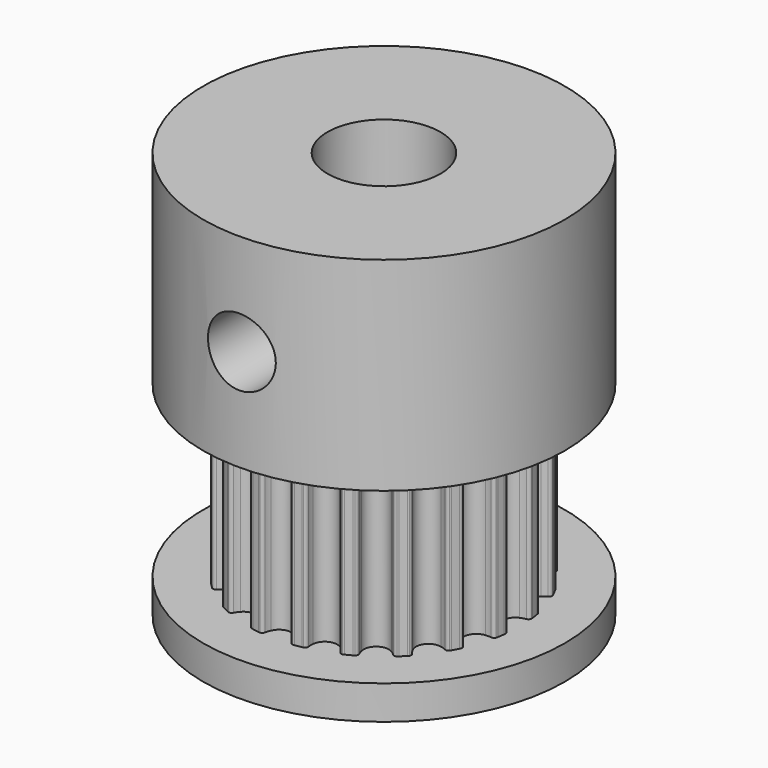
from build123d import *

# Parameters (mm, degrees)
F1_DEPTH  = 7.5
F2_R      = 8
F3_DEPTH  = 9
F4_R      = 8
F5_DEPTH  = 1.5
F6_R      = 2.5
F7_DEPTH  = 18.001
F8_R      = 1.5
F9_DEPTH  = 8.001
F10_R     = 1.5
F11_DEPTH = 10


with BuildPart() as f1:
    # F0 (on Top) → F1 (new body)
    with BuildSketch(Plane.XY):
        with BuildLine():
            ThreePointArc((-0.5137469529, -5.5950260293), (0, -5.25), (0.5137469529, -5.5950260293))
            ThreePointArc((0.5137469529, -5.5950260293), (0.5592692601, -5.7125893356), (0.5896381917, -5.8349459432))
            ThreePointArc((0.5896381917, -5.8349459432), (0.634011817, -5.9169199806), (0.718236871, -5.9568562008))
            ThreePointArc((0.718236871, -5.9568562008), (0.7555100891, -5.952243653), (0.7927537045, -5.9473978818))
            ThreePointArc((0.7927537045, -5.9473978818), (0.9386067902, -5.9261300436), (1.0838934413, -5.9012858775))
            ThreePointArc((1.0838934413, -5.9012858775), (1.1208116501, -5.8943855698), (1.1576859427, -5.8872543055))
            ThreePointArc((1.1576859427, -5.8872543055), (1.2254477584, -5.82324573), (1.2423182132, -5.7315715833))
            ThreePointArc((1.2423182132, -5.7315715833), (1.2333905124, -5.6058190183), (1.2403557397, -5.4799425032))
            ThreePointArc((1.2403557397, -5.4799425032), (1.6223392205, -4.9930467105), (2.2175605143, -5.1624294247))
            ThreePointArc((2.2175605143, -5.1624294247), (2.2971838607, -5.2601716067), (2.3638767022, -5.3671551397))
            ThreePointArc((2.3638767022, -5.3671551397), (2.4314098983, -5.4314048778), (2.5238536555, -5.4433595073))
            ThreePointArc((2.5238536555, -5.4433595073), (2.5578772368, -5.4274546558), (2.5918005942, -5.4113371434))
            ThreePointArc((2.5918005942, -5.4113371434), (2.7239429984, -5.3460391451), (2.8544415451, -5.2775148949))
            ThreePointArc((2.8544415451, -5.2775148949), (2.8874205358, -5.2595439583), (2.9202863902, -5.2413669399))
            ThreePointArc((2.9202863902, -5.2413669399), (2.964951969, -5.1595516144), (2.9526678557, -5.0671510626))
            ThreePointArc((2.9526678557, -5.0671510626), (2.905317428, -4.9503120775), (2.8730437705, -4.828444024))
            ThreePointArc((2.8730437705, -4.828444024), (3.0858725745, -4.2473392205), (3.7043038019, -4.2244982593))
            ThreePointArc((3.7043038019, -4.2244982593), (3.8102340997, -4.2928516312), (3.906722491, -4.373989796))
            ThreePointArc((3.906722491, -4.373989796), (3.9908046381, -4.4142260228), (4.0824180595, -4.3970288591))
            ThreePointArc((4.0824180595, -4.3970288591), (4.1098615388, -4.3713885816), (4.1371439837, -4.3455770225))
            ThreePointArc((4.1371439837, -4.3455770225), (4.2426406871, -4.2426406871), (4.3455770225, -4.1371439837))
            ThreePointArc((4.3455770225, -4.1371439837), (4.3713885816, -4.1098615388), (4.3970288591, -4.0824180595))
            ThreePointArc((4.3970288591, -4.0824180595), (4.4142260228, -3.9908046381), (4.373989796, -3.906722491))
            ThreePointArc((4.373989796, -3.906722491), (4.2928516312, -3.8102340997), (4.2244982593, -3.7043038019))
            ThreePointArc((4.2244982593, -3.7043038019), (4.2473392205, -3.0858725745), (4.828444024, -2.8730437705))
            ThreePointArc((4.828444024, -2.8730437705), (4.9503120775, -2.905317428), (5.0671510626, -2.9526678557))
            ThreePointArc((5.0671510626, -2.9526678557), (5.1595516144, -2.964951969), (5.2413669399, -2.9202863902))
            ThreePointArc((5.2413669399, -2.9202863902), (5.2595439583, -2.8874205358), (5.2775148949, -2.8544415451))
            ThreePointArc((5.2775148949, -2.8544415451), (5.3460391451, -2.7239429984), (5.4113371434, -2.5918005942))
            ThreePointArc((5.4113371434, -2.5918005942), (5.4432427829, -2.4673716464), (5.3671551397, -2.3638767022))
            ThreePointArc((5.3671551397, -2.3638767022), (5.2601716067, -2.2971838607), (5.1624294247, -2.2175605143))
            ThreePointArc((5.1624294247, -2.2175605143), (4.9930467105, -1.6223392205), (5.4799425032, -1.2403557397))
            ThreePointArc((5.4799425032, -1.2403557397), (5.6058190183, -1.2333905124), (5.7315715833, -1.2423182132))
            ThreePointArc((5.7315715833, -1.2423182132), (5.82324573, -1.2254477584), (5.8872543055, -1.1576859427))
            ThreePointArc((5.8872543055, -1.1576859427), (5.8943855698, -1.1208116501), (5.9012858775, -1.0838934413))
            ThreePointArc((5.9012858775, -1.0838934413), (5.9261300436, -0.9386067902), (5.9473978818, -0.7927537045))
            ThreePointArc((5.9473978818, -0.7927537045), (5.952243653, -0.7555100891), (5.9568562008, -0.718236871))
            ThreePointArc((5.9568562008, -0.718236871), (5.9169199806, -0.634011817), (5.8349459432, -0.5896381917))
            ThreePointArc((5.8349459432, -0.5896381917), (5.7125893356, -0.5592692601), (5.5950260293, -0.5137469529))
            ThreePointArc((5.5950260293, -0.5137469529), (5.25, 0), (5.5950260293, 0.5137469529))
            ThreePointArc((5.5950260293, 0.5137469529), (5.7125893356, 0.5592692601), (5.8349459432, 0.5896381917))
            ThreePointArc((5.8349459432, 0.5896381917), (5.9169199806, 0.634011817), (5.9568562008, 0.718236871))
            ThreePointArc((5.9568562008, 0.718236871), (5.952243653, 0.7555100891), (5.9473978818, 0.7927537045))
            ThreePointArc((5.9473978818, 0.7927537045), (5.9261300436, 0.9386067902), (5.9012858775, 1.0838934413))
            ThreePointArc((5.9012858775, 1.0838934413), (5.8943855698, 1.1208116501), (5.8872543055, 1.1576859427))
            ThreePointArc((5.8872543055, 1.1576859427), (5.82324573, 1.2254477584), (5.7315715833, 1.2423182132))
            ThreePointArc((5.7315715833, 1.2423182132), (5.6058190183, 1.2333905124), (5.4799425032, 1.2403557397))
            ThreePointArc((5.4799425032, 1.2403557397), (4.9930467105, 1.6223392205), (5.1624294247, 2.2175605143))
            ThreePointArc((5.1624294247, 2.2175605143), (5.2601716067, 2.2971838607), (5.3671551397, 2.3638767022))
            ThreePointArc((5.3671551397, 2.3638767022), (5.4314048778, 2.4314098983), (5.4433595073, 2.5238536555))
            ThreePointArc((5.4433595073, 2.5238536555), (5.4274546558, 2.5578772368), (5.4113371434, 2.5918005942))
            ThreePointArc((5.4113371434, 2.5918005942), (5.3460391451, 2.7239429984), (5.2775148949, 2.8544415451))
            ThreePointArc((5.2775148949, 2.8544415451), (5.2595439583, 2.8874205358), (5.2413669399, 2.9202863902))
            ThreePointArc((5.2413669399, 2.9202863902), (5.1595516144, 2.964951969), (5.0671510626, 2.9526678557))
            ThreePointArc((5.0671510626, 2.9526678557), (4.9503120775, 2.905317428), (4.828444024, 2.8730437705))
            ThreePointArc((4.828444024, 2.8730437705), (4.2473392205, 3.0858725745), (4.2244982593, 3.7043038019))
            ThreePointArc((4.2244982593, 3.7043038019), (4.2928516312, 3.8102340997), (4.373989796, 3.906722491))
            ThreePointArc((4.373989796, 3.906722491), (4.4142260228, 3.9908046381), (4.3970288591, 4.0824180595))
            ThreePointArc((4.3970288591, 4.0824180595), (4.3713885816, 4.1098615388), (4.3455770225, 4.1371439837))
            ThreePointArc((4.3455770225, 4.1371439837), (4.2426406871, 4.2426406871), (4.1371439837, 4.3455770225))
            ThreePointArc((4.1371439837, 4.3455770225), (4.1098615388, 4.3713885816), (4.0824180595, 4.3970288591))
            ThreePointArc((4.0824180595, 4.3970288591), (3.9908046381, 4.4142260228), (3.906722491, 4.373989796))
            ThreePointArc((3.906722491, 4.373989796), (3.8102340997, 4.2928516312), (3.7043038019, 4.2244982593))
            ThreePointArc((3.7043038019, 4.2244982593), (3.0858725745, 4.2473392205), (2.8730437705, 4.828444024))
            ThreePointArc((2.8730437705, 4.828444024), (2.905317428, 4.9503120775), (2.9526678557, 5.0671510626))
            ThreePointArc((2.9526678557, 5.0671510626), (2.964951969, 5.1595516144), (2.9202863902, 5.2413669399))
            ThreePointArc((2.9202863902, 5.2413669399), (2.8874205358, 5.2595439583), (2.8544415451, 5.2775148949))
            ThreePointArc((2.8544415451, 5.2775148949), (2.7239429984, 5.3460391451), (2.5918005942, 5.4113371434))
            ThreePointArc((2.5918005942, 5.4113371434), (2.5578772368, 5.4274546558), (2.5238536555, 5.4433595073))
            ThreePointArc((2.5238536555, 5.4433595073), (2.4314098983, 5.4314048778), (2.3638767022, 5.3671551397))
            ThreePointArc((2.3638767022, 5.3671551397), (2.2971838607, 5.2601716067), (2.2175605143, 5.1624294247))
            ThreePointArc((2.2175605143, 5.1624294247), (1.6223392205, 4.9930467105), (1.2403557397, 5.4799425032))
            ThreePointArc((1.2403557397, 5.4799425032), (1.2333905124, 5.6058190183), (1.2423182132, 5.7315715833))
            ThreePointArc((1.2423182132, 5.7315715833), (1.2254477584, 5.82324573), (1.1576859427, 5.8872543055))
            ThreePointArc((1.1576859427, 5.8872543055), (1.1208116501, 5.8943855698), (1.0838934413, 5.9012858775))
            ThreePointArc((1.0838934413, 5.9012858775), (0.9386067902, 5.9261300436), (0.7927537045, 5.9473978818))
            ThreePointArc((0.7927537045, 5.9473978818), (0.7555100891, 5.952243653), (0.718236871, 5.9568562008))
            ThreePointArc((0.718236871, 5.9568562008), (0.634011817, 5.9169199806), (0.5896381917, 5.8349459432))
            ThreePointArc((0.5896381917, 5.8349459432), (0.5592692601, 5.7125893356), (0.5137469529, 5.5950260293))
            ThreePointArc((0.5137469529, 5.5950260293), (0, 5.25), (-0.5137469529, 5.5950260293))
            ThreePointArc((-0.5137469529, 5.5950260293), (-0.5592692601, 5.7125893356), (-0.5896381917, 5.8349459432))
            ThreePointArc((-0.5896381917, 5.8349459432), (-0.634011817, 5.9169199806), (-0.718236871, 5.9568562008))
            ThreePointArc((-0.718236871, 5.9568562008), (-0.7555100891, 5.952243653), (-0.7927537045, 5.9473978818))
            ThreePointArc((-0.7927537045, 5.9473978818), (-0.9386067902, 5.9261300436), (-1.0838934413, 5.9012858775))
            ThreePointArc((-1.0838934413, 5.9012858775), (-1.1208116501, 5.8943855698), (-1.1576859427, 5.8872543055))
            ThreePointArc((-1.1576859427, 5.8872543055), (-1.2254477584, 5.82324573), (-1.2423182132, 5.7315715833))
            ThreePointArc((-1.2423182132, 5.7315715833), (-1.2333905124, 5.6058190183), (-1.2403557397, 5.4799425032))
            ThreePointArc((-1.2403557397, 5.4799425032), (-1.6223392205, 4.9930467105), (-2.2175605143, 5.1624294247))
            ThreePointArc((-2.2175605143, 5.1624294247), (-2.2971838607, 5.2601716067), (-2.3638767022, 5.3671551397))
            ThreePointArc((-2.3638767022, 5.3671551397), (-2.4314098983, 5.4314048778), (-2.5238536555, 5.4433595073))
            ThreePointArc((-2.5238536555, 5.4433595073), (-2.5578772368, 5.4274546558), (-2.5918005942, 5.4113371434))
            ThreePointArc((-2.5918005942, 5.4113371434), (-2.7239429984, 5.3460391451), (-2.8544415451, 5.2775148949))
            ThreePointArc((-2.8544415451, 5.2775148949), (-2.8874205358, 5.2595439583), (-2.9202863902, 5.2413669399))
            ThreePointArc((-2.9202863902, 5.2413669399), (-2.964951969, 5.1595516144), (-2.9526678557, 5.0671510626))
            ThreePointArc((-2.9526678557, 5.0671510626), (-2.905317428, 4.9503120775), (-2.8730437705, 4.828444024))
            ThreePointArc((-2.8730437705, 4.828444024), (-3.0858725745, 4.2473392205), (-3.7043038019, 4.2244982593))
            ThreePointArc((-3.7043038019, 4.2244982593), (-3.8102340997, 4.2928516312), (-3.906722491, 4.373989796))
            ThreePointArc((-3.906722491, 4.373989796), (-3.9908046381, 4.4142260228), (-4.0824180595, 4.3970288591))
            ThreePointArc((-4.0824180595, 4.3970288591), (-4.1098615388, 4.3713885816), (-4.1371439837, 4.3455770225))
            ThreePointArc((-4.1371439837, 4.3455770225), (-4.2426406871, 4.2426406871), (-4.3455770225, 4.1371439837))
            ThreePointArc((-4.3455770225, 4.1371439837), (-4.3713885816, 4.1098615388), (-4.3970288591, 4.0824180595))
            ThreePointArc((-4.3970288591, 4.0824180595), (-4.4142260228, 3.9908046381), (-4.373989796, 3.906722491))
            ThreePointArc((-4.373989796, 3.906722491), (-4.2928516312, 3.8102340997), (-4.2244982593, 3.7043038019))
            ThreePointArc((-4.2244982593, 3.7043038019), (-4.2473392205, 3.0858725745), (-4.828444024, 2.8730437705))
            ThreePointArc((-4.828444024, 2.8730437705), (-4.9503120775, 2.905317428), (-5.0671510626, 2.9526678557))
            ThreePointArc((-5.0671510626, 2.9526678557), (-5.1595516144, 2.964951969), (-5.2413669399, 2.9202863902))
            ThreePointArc((-5.2413669399, 2.9202863902), (-5.2595439583, 2.8874205358), (-5.2775148949, 2.8544415451))
            ThreePointArc((-5.2775148949, 2.8544415451), (-5.3460391451, 2.7239429984), (-5.4113371434, 2.5918005942))
            ThreePointArc((-5.4113371434, 2.5918005942), (-5.4274546558, 2.5578772368), (-5.4433595073, 2.5238536555))
            ThreePointArc((-5.4433595073, 2.5238536555), (-5.4314048778, 2.4314098983), (-5.3671551397, 2.3638767022))
            ThreePointArc((-5.3671551397, 2.3638767022), (-5.2601716067, 2.2971838607), (-5.1624294247, 2.2175605143))
            ThreePointArc((-5.1624294247, 2.2175605143), (-4.9930467105, 1.6223392205), (-5.4799425032, 1.2403557397))
            ThreePointArc((-5.4799425032, 1.2403557397), (-5.6058190183, 1.2333905124), (-5.7315715833, 1.2423182132))
            ThreePointArc((-5.7315715833, 1.2423182132), (-5.82324573, 1.2254477584), (-5.8872543055, 1.1576859427))
            ThreePointArc((-5.8872543055, 1.1576859427), (-5.8943855698, 1.1208116501), (-5.9012858775, 1.0838934413))
            ThreePointArc((-5.9012858775, 1.0838934413), (-5.9261300436, 0.9386067902), (-5.9473978818, 0.7927537045))
            ThreePointArc((-5.9473978818, 0.7927537045), (-5.952243653, 0.7555100891), (-5.9568562008, 0.718236871))
            ThreePointArc((-5.9568562008, 0.718236871), (-5.9169199806, 0.634011817), (-5.8349459432, 0.5896381917))
            ThreePointArc((-5.8349459432, 0.5896381917), (-5.7125893356, 0.5592692601), (-5.5950260293, 0.5137469529))
            ThreePointArc((-5.5950260293, 0.5137469529), (-5.25, 0), (-5.5950260293, -0.5137469529))
            ThreePointArc((-5.5950260293, -0.5137469529), (-5.7125893356, -0.5592692601), (-5.8349459432, -0.5896381917))
            ThreePointArc((-5.8349459432, -0.5896381917), (-5.9169199806, -0.634011817), (-5.9568562008, -0.718236871))
            ThreePointArc((-5.9568562008, -0.718236871), (-5.952243653, -0.7555100891), (-5.9473978818, -0.7927537045))
            ThreePointArc((-5.9473978818, -0.7927537045), (-5.9261300436, -0.9386067902), (-5.9012858775, -1.0838934413))
            ThreePointArc((-5.9012858775, -1.0838934413), (-5.8943855698, -1.1208116501), (-5.8872543055, -1.1576859427))
            ThreePointArc((-5.8872543055, -1.1576859427), (-5.82324573, -1.2254477584), (-5.7315715833, -1.2423182132))
            ThreePointArc((-5.7315715833, -1.2423182132), (-5.6058190183, -1.2333905124), (-5.4799425032, -1.2403557397))
            ThreePointArc((-5.4799425032, -1.2403557397), (-4.9930467105, -1.6223392205), (-5.1624294247, -2.2175605143))
            ThreePointArc((-5.1624294247, -2.2175605143), (-5.2601716067, -2.2971838607), (-5.3671551397, -2.3638767022))
            ThreePointArc((-5.3671551397, -2.3638767022), (-5.4314048778, -2.4314098983), (-5.4433595073, -2.5238536555))
            ThreePointArc((-5.4433595073, -2.5238536555), (-5.4274546558, -2.5578772368), (-5.4113371434, -2.5918005942))
            ThreePointArc((-5.4113371434, -2.5918005942), (-5.3460391451, -2.7239429984), (-5.2775148949, -2.8544415451))
            ThreePointArc((-5.2775148949, -2.8544415451), (-5.2595439583, -2.8874205358), (-5.2413669399, -2.9202863902))
            ThreePointArc((-5.2413669399, -2.9202863902), (-5.1595516144, -2.964951969), (-5.0671510626, -2.9526678557))
            ThreePointArc((-5.0671510626, -2.9526678557), (-4.9503120775, -2.905317428), (-4.828444024, -2.8730437705))
            ThreePointArc((-4.828444024, -2.8730437705), (-4.2473392205, -3.0858725745), (-4.2244982593, -3.7043038019))
            ThreePointArc((-4.2244982593, -3.7043038019), (-4.2928516312, -3.8102340997), (-4.373989796, -3.906722491))
            ThreePointArc((-4.373989796, -3.906722491), (-4.4142260228, -3.9908046381), (-4.3970288591, -4.0824180595))
            ThreePointArc((-4.3970288591, -4.0824180595), (-4.3713885816, -4.1098615388), (-4.3455770225, -4.1371439837))
            ThreePointArc((-4.3455770225, -4.1371439837), (-4.2426406871, -4.2426406871), (-4.1371439837, -4.3455770225))
            ThreePointArc((-4.1371439837, -4.3455770225), (-4.1098615388, -4.3713885816), (-4.0824180595, -4.3970288591))
            ThreePointArc((-4.0824180595, -4.3970288591), (-3.9908046381, -4.4142260228), (-3.906722491, -4.373989796))
            ThreePointArc((-3.906722491, -4.373989796), (-3.8102340997, -4.2928516312), (-3.7043038019, -4.2244982593))
            ThreePointArc((-3.7043038019, -4.2244982593), (-3.0858725745, -4.2473392205), (-2.8730437705, -4.828444024))
            ThreePointArc((-2.8730437705, -4.828444024), (-2.905317428, -4.9503120775), (-2.9526678557, -5.0671510626))
            ThreePointArc((-2.9526678557, -5.0671510626), (-2.964951969, -5.1595516144), (-2.9202863902, -5.2413669399))
            ThreePointArc((-2.9202863902, -5.2413669399), (-2.8874205358, -5.2595439583), (-2.8544415451, -5.2775148949))
            ThreePointArc((-2.8544415451, -5.2775148949), (-2.7239429984, -5.3460391451), (-2.5918005942, -5.4113371434))
            ThreePointArc((-2.5918005942, -5.4113371434), (-2.5578772368, -5.4274546558), (-2.5238536555, -5.4433595073))
            ThreePointArc((-2.5238536555, -5.4433595073), (-2.4314098983, -5.4314048778), (-2.3638767022, -5.3671551397))
            ThreePointArc((-2.3638767022, -5.3671551397), (-2.2971838607, -5.2601716067), (-2.2175605143, -5.1624294247))
            ThreePointArc((-2.2175605143, -5.1624294247), (-1.6223392205, -4.9930467105), (-1.2403557397, -5.4799425032))
            ThreePointArc((-1.2403557397, -5.4799425032), (-1.2333905124, -5.6058190183), (-1.2423182132, -5.7315715833))
            ThreePointArc((-1.2423182132, -5.7315715833), (-1.2254477584, -5.82324573), (-1.1576859427, -5.8872543055))
            ThreePointArc((-1.1576859427, -5.8872543055), (-1.1208116501, -5.8943855698), (-1.0838934413, -5.9012858775))
            ThreePointArc((-1.0838934413, -5.9012858775), (-0.9386067902, -5.9261300436), (-0.7927537045, -5.9473978818))
            ThreePointArc((-0.7927537045, -5.9473978818), (-0.7555100891, -5.952243653), (-0.718236871, -5.9568562008))
            ThreePointArc((-0.718236871, -5.9568562008), (-0.634011817, -5.9169199806), (-0.5896381917, -5.8349459432))
            ThreePointArc((-0.5896381917, -5.8349459432), (-0.5592692601, -5.7125893356), (-0.5137469529, -5.5950260293))
        make_face()
    extrude(amount=F1_DEPTH)

    # F2 (on face) → F3 (join)
    with BuildSketch(Plane.XY.offset(7.5)):
        Circle(F2_R)
    extrude(amount=F3_DEPTH)

    # F4 (on face) → F5 (join)
    with BuildSketch(Plane(origin=(0, 0, 0), x_dir=(1, 0, 0), z_dir=(0, 0, -1))):
        Circle(F4_R)
    extrude(amount=F5_DEPTH)

    # F6 (on face) → F7 (cut, through all)
    with BuildSketch(Plane(origin=(0, 0, -1.5), x_dir=(1, 0, 0), z_dir=(0, 0, -1))):
        Circle(F6_R)
    extrude(amount=-F7_DEPTH, mode=Mode.SUBTRACT)

    # F8 (on Right) → F9 (cut, through all)
    with BuildSketch(Plane.YZ):
        with Locations((0, 12)):
            Circle(F8_R)
    extrude(amount=-F9_DEPTH, mode=Mode.SUBTRACT)

    # F10 (on Front) → F11 (cut)
    with BuildSketch(Plane.XZ):
        with Locations((0, 12)):
            Circle(F10_R)
    extrude(amount=F11_DEPTH, mode=Mode.SUBTRACT)


solid = f1.part
